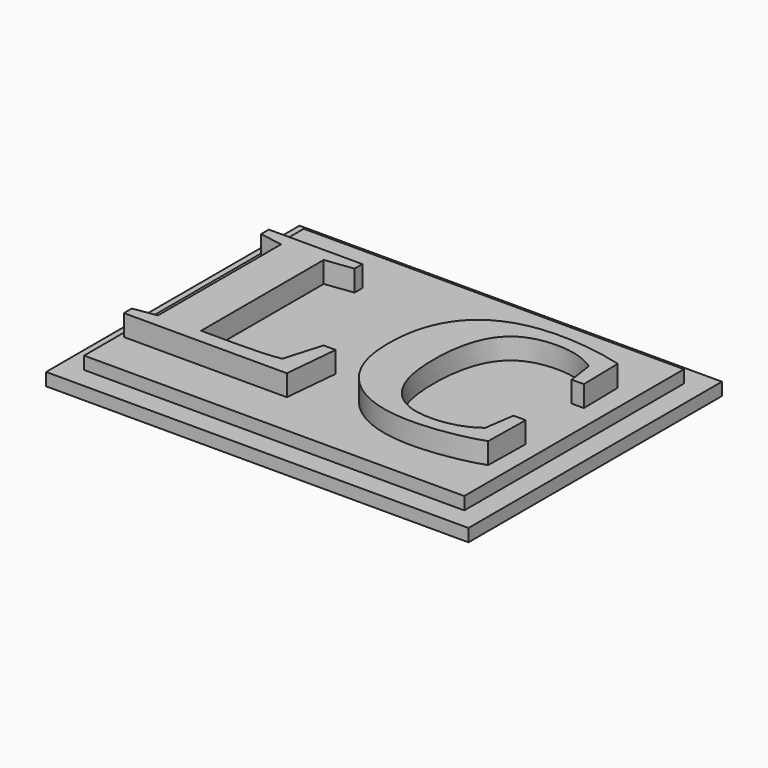
from build123d import *

# Parameters (mm, degrees)
F0_W         = 40
F0_H         = 30
F1_DEPTH     = 1.2
F2_W         = 36
F2_H         = 26
F3_DEPTH     = 1.2
F4_TEXT_SIZE = 26.1728956038
F5_DEPTH     = 2


# Not quite as in the source:
# - Text() gives the source's letters only with a copy of the font that has no kerning and outlines rounded to 1/6400 em; it was checked with that copy


with BuildPart() as f1:
    # F0 (on Top) → F1 (new body)
    with BuildSketch(Plane.XY):
        with Locations((20, 15)):
            Rectangle(F0_W, F0_H)
    extrude(amount=F1_DEPTH)

    # F2 (on face) → F3 (join)
    with BuildSketch(Plane.XY.offset(1.2)):
        with Locations((20, 15)):
            Rectangle(F2_W, F2_H)
    extrude(amount=F3_DEPTH)

    # F4 (on face) → F5 (join)
    with BuildSketch(Plane.XY.offset(2.4)):
        with Locations((2, 6.1555151653)):
            Text('LC', F4_TEXT_SIZE, font='Tinos', font_style=FontStyle.BOLD, text_align=(TextAlign.LEFT, TextAlign.BOTTOM))
    extrude(amount=F5_DEPTH)


solid = f1.part
